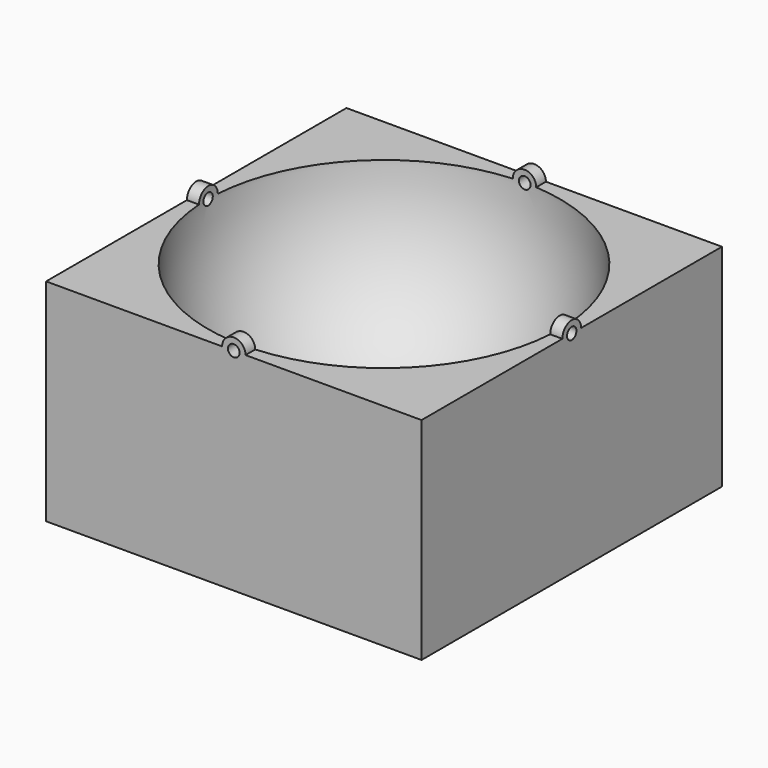
from build123d import *

# Parameters (mm, degrees)
F1_DEPTH      = 203.2
F1_DEPTH_BACK = 203.2
F4_DEPTH      = 406.4
F5_R          = 6.35
F6_DEPTH      = 406.4


# Not quite as in the source:
# - a feature names something its author has since deleted; it is built from what else it names


with BuildPart() as f1:
    # F0 (on Front) → F1 (new body, two sides)
    with BuildSketch(Plane.XZ) as f1_sk:
        with BuildLine():
            Line((203.2, 0), (12.7, 0))
            ThreePointArc((12.7, 0), (0, -12.7), (-12.7, 0))
            Line((-12.7, 0), (-203.2, 0))
            Line((-203.2, 0), (-203.2, -228.6))
            Line((-203.2, -228.6), (203.2, -228.6))
            Line((203.2, -228.6), (203.2, 0))
        make_face()
        with BuildLine():
            Line((12.7, 0), (6.35, 0))
            ThreePointArc((6.35, 0), (0, -6.35), (-6.35, 0))
            Line((-6.35, 0), (-12.7, 0))
            ThreePointArc((-12.7, 0), (0, -12.7), (12.7, 0))
        make_face()
        with BuildLine():
            ThreePointArc((-6.35, 0), (0, 6.35), (6.35, 0))
            Line((6.35, 0), (12.7, 0))
            ThreePointArc((12.7, 0), (0, 12.7), (-12.7, 0))
            Line((-12.7, 0), (-6.35, 0))
        make_face()
    extrude(amount=F1_DEPTH)
    extrude(f1_sk.sketch, amount=-F1_DEPTH_BACK)

    # F3 (on face) → F4 (join)
    with BuildSketch(Plane.YZ.offset(203.2)):
        with BuildLine():
            Line((-12.7, 0), (12.7, 0))
            ThreePointArc((12.7, 0), (0, 12.7), (-12.7, 0))
        make_face()
        with BuildLine():
            ThreePointArc((-12.7, 0), (0, -12.7), (12.7, 0))
            Line((12.7, 0), (-12.7, 0))
        make_face()
    extrude(amount=-F4_DEPTH)

    # F5 (on face) → F6 (cut)
    with BuildSketch(Plane.YZ.offset(203.2)):
        Circle(F5_R)
    extrude(amount=-F6_DEPTH, mode=Mode.SUBTRACT)

    # F2 (on Front) → F7 (revolve, cut)
    with BuildSketch(Plane.XZ):
        with BuildLine():
            Line((0, 190.5), (0, -190.5))
            ThreePointArc((0, -190.5), (190.5, 0), (0, 190.5))
        make_face()
    revolve(axis=Axis((0, 0, 0), (0, 0, -1)), mode=Mode.SUBTRACT)


solid = f1.part
